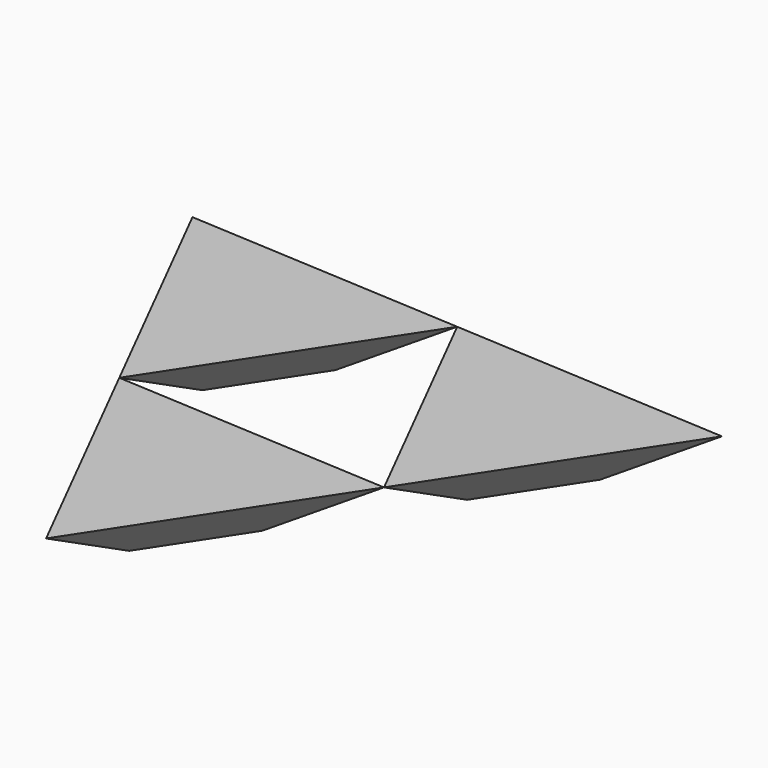
from build123d import *

# Parameters (mm, degrees)
F1_DEPTH  = 50.8
F2_SIZE   = 101.59999
F2_2_SIZE = 101.59999
F2_3_SIZE = 101.59999


# Not quite as in the source:
# - a fillet or chamfer is up to 0.001 mm smaller than in the source, because OpenCascade refuses the exact size


with BuildPart() as f1:
    # F0 (on Top) → F1 (new body, symmetric)
    with BuildSketch(Plane.XY):
        Polygon((280.3652053341, -183.6145129428), (598.3948707581, 301.9922673702), (18.832230045, 334.6106466279), align=None)
    extrude(amount=F1_DEPTH, both=True)

    # F2 (size 101.6 in the source; OpenCascade refuses exactly that, so slightly less here)
    f2_edges = [f1.edges().sort_by_distance(p)[0] for p in [
        (308.61355, 318.301457, -50.8),
        (439.380038, 59.188877, -50.8),
        (149.598718, 75.498067, -50.8),
    ]]
    chamfer(f2_edges, length=F2_SIZE)


with BuildPart() as f1b:
    # F0 (on Top) → F1, piece 2 (new body, symmetric)
    with BuildSketch(Plane.XY):
        Polygon((-37.66446009, -669.2212932559), (280.3652053341, -183.6145129428), (-299.197435379, -150.9961336851), align=None)
    extrude(amount=F1_DEPTH, both=True)

    # F2#2 (size 101.6 in the source; OpenCascade refuses exactly that, so slightly less here)
    f2_2_edges = [f1b.edges().sort_by_distance(p)[0] for p in [
        (-9.416115, -167.305323, -50.8),
        (121.350373, -426.417903, -50.8),
        (-168.430948, -410.108713, -50.8),
    ]]
    chamfer(f2_2_edges, length=F2_2_SIZE)


with BuildPart() as f1c:
    # F0 (on Top) → F1, piece 3 (new body, symmetric)
    with BuildSketch(Plane.XY):
        Polygon((-299.197435379, -150.9961336851), (18.832230045, 334.6106466279), (-560.7304106681, 367.2290258857), align=None)
    extrude(amount=F1_DEPTH, both=True)

    # F2#3 (size 101.6 in the source; OpenCascade refuses exactly that, so slightly less here)
    f2_3_edges = [f1c.edges().sort_by_distance(p)[0] for p in [
        (-429.963923, 108.116446, -50.8),
        (-270.94909, 350.919836, -50.8),
        (-140.182603, 91.807256, -50.8),
    ]]
    chamfer(f2_3_edges, length=F2_3_SIZE)


solid = Compound([f1.part, f1b.part, f1c.part])
